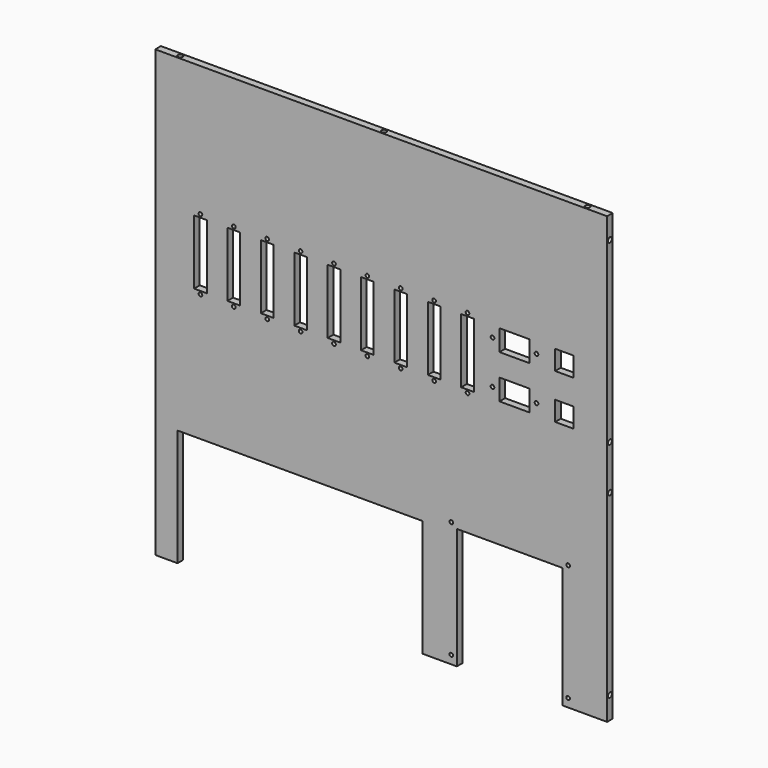
from build123d import *

# Parameters (mm, degrees)
F0_W           = 11.4
F0_H           = 57.9
F0_W_2         = 27
F0_H_2         = 18.9
F0_W_3         = 16.7
F0_H_3         = 17.6
F1_DEPTH       = 3.175
F5_D           = 4.4
F5_DEPTH       = 12
F5_TIP         = 1.3218933619
F6_D           = 4.4
F6_DEPTH       = 12
F6_TIP         = 1.3218933619
F6_ON_F4_D     = 4.4
F6_ON_F4_DEPTH = 12
F6_ON_F4_TIP   = 1.3218933619
F8_D           = 3.3


# Not quite as in the source:
# - a feature names something its author has since deleted; it is built from what else it names


with BuildPart() as f1:
    # F0 (on Front) → F1 (new body, symmetric)
    with BuildSketch(Plane.XZ):
        Polygon((163, -200), (203, -200), (203, 200), (-203, 200), (-203, -200), (-183, -200), (-183, -95), (37, -95), (37, -200), (68, -200), (68, -91.22133255), (163, -91.22133255), align=None)
        with Locations((-162.4, 51.05)):
            Rectangle(F0_W, F0_H, mode=Mode.SUBTRACT)
        with Locations((-132.4, 51.05)):
            Rectangle(F0_W, F0_H, mode=Mode.SUBTRACT)
        with Locations((-102.4, 51.05)):
            Rectangle(F0_W, F0_H, mode=Mode.SUBTRACT)
        with Locations((-72.4, 51.05)):
            Rectangle(F0_W, F0_H, mode=Mode.SUBTRACT)
        with Locations((-42.4, 51.05)):
            Rectangle(F0_W, F0_H, mode=Mode.SUBTRACT)
        with Locations((-12.4, 51.05)):
            Rectangle(F0_W, F0_H, mode=Mode.SUBTRACT)
        with Locations((17.6, 51.05)):
            Rectangle(F0_W, F0_H, mode=Mode.SUBTRACT)
        with Locations((47.6, 51.05)):
            Rectangle(F0_W, F0_H, mode=Mode.SUBTRACT)
        with Locations((77.6, 51.05)):
            Rectangle(F0_W, F0_H, mode=Mode.SUBTRACT)
        with Locations((119.8, 31.55)):
            Rectangle(F0_W_2, F0_H_2, mode=Mode.SUBTRACT)
        with Locations((164.65, 30.9)):
            Rectangle(F0_W_3, F0_H_3, mode=Mode.SUBTRACT)
        with Locations((119.8, 70.55)):
            Rectangle(F0_W_2, F0_H_2, mode=Mode.SUBTRACT)
        with Locations((164.65, 71.2)):
            Rectangle(F0_W_3, F0_H_3, mode=Mode.SUBTRACT)
    extrude(amount=F1_DEPTH, both=True)

    # F5
    with Locations(Plane.XY.offset(200)):
        with Locations((-183, 0), (0, 0), (183, 0)):
            Hole(F5_D / 2, depth=F5_DEPTH)
            with Locations((0, 0, -(F5_DEPTH + F5_TIP / 2))):  # 118° drill point
                Cone(0, F5_D / 2, F5_TIP, mode=Mode.SUBTRACT)

    # F6
    with Locations(Plane(origin=(-203, 0, 0), x_dir=(0, -1, 0), z_dir=(-1, 0, 0))):
        with Locations((0, -180), (0, -20), (0, 20), (0, 180)):
            Hole(F6_D / 2, depth=F6_DEPTH)
            with Locations((0, 0, -(F6_DEPTH + F6_TIP / 2))):  # 118° drill point
                Cone(0, F6_D / 2, F6_TIP, mode=Mode.SUBTRACT)

    # F6 on F4
    with Locations(Plane.YZ.offset(203)):
        with Locations((0, -180), (0, -20), (0, 20), (0, 180)):
            Hole(F6_ON_F4_D / 2, depth=F6_ON_F4_DEPTH)
            with Locations((0, 0, -(F6_ON_F4_DEPTH + F6_ON_F4_TIP / 2))):  # 118° drill point
                Cone(0, F6_ON_F4_D / 2, F6_ON_F4_TIP, mode=Mode.SUBTRACT)

    # F8 (through all)
    with Locations(Plane.XZ.offset(3.175)):
        with Locations((63, -87.5), (168, -87.5), (168, -192.5), (63, -192.5), (77.6, 82.8), (47.6, 82.8), (77.6, 19.3), (47.6, 19.3), (17.6, 19.3), (17.6, 82.8), (-12.4, 82.8), (-12.4, 19.3), (-42.4, 19.3), (-42.4, 82.8), (-72.4, 82.8), (-72.4, 19.3), (-102.4, 19.3), (-102.4, 82.8), (-132.4, 82.8), (-132.4, 19.3), (-162.4, 19.3), (-162.4, 82.8), (139.55, 70.55), (100.05, 70.55), (100.05, 31.55), (139.55, 31.55)):
            Hole(F8_D / 2)


solid = f1.part
